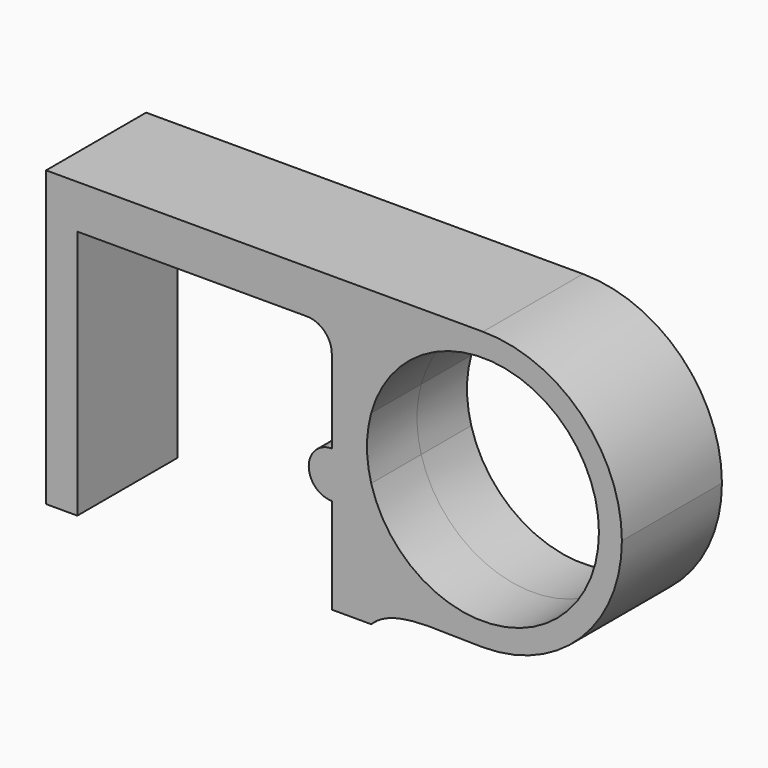
from build123d import *

# Parameters (mm, degrees)
F1_DEPTH = 5


with BuildPart() as f1:
    # F0 (on Front) → F1 (new body, symmetric)
    with BuildSketch(Plane.XZ):
        with BuildLine():
            Line((-24.5694083333, 31.5104130507), (-50.5694083333, 31.5104130507))
            Line((-50.5694083333, 31.5104130507), (-50.5694083333, 8.0104130507))
            Line((-50.5694083333, 8.0104130507), (-48.0694083333, 8.0104130507))
            Line((-48.0694083333, 8.0104130507), (-48.0694083333, 28.0104130507))
            Line((-48.0694083333, 28.0104130507), (-29.7194083333, 28.0104130507))
            ThreePointArc((-29.7194083333, 28.0104130507), (-28.3051947709, 27.424626613), (-27.7194083333, 26.0104130507))
            Line((-27.7194083333, 26.0104130507), (-27.7194083333, 19.3554483443))
            Line((-27.7194083333, 19.3554483443), (-27.7194083333, 15.665377757))
            Line((-27.7194083333, 15.665377757), (-27.7194083333, 8.0104130507))
            Line((-27.7194083333, 8.0104130507), (-24.5694083333, 8.0104130507))
            Line((-24.5694083333, 8.0104130507), (-24.5694083333, 13.8020069146))
            ThreePointArc((-24.5694083333, 13.8020069146), (-26.7411284149, 20.4004295021), (-24.5694083333, 26.9988520897))
            Line((-24.5694083333, 26.9988520897), (-24.5694083333, 31.5104130507))
        make_face()
        with BuildLine():
            ThreePointArc((-15.6311448663, 31.5104130507), (-20.6373094688, 30.3185971969), (-24.5694083333, 26.9988520897))
            Line((-24.5694083333, 26.9988520897), (-24.5694083333, 22.8769333271))
            ThreePointArc((-24.5694083333, 22.8769333271), (-14.3814986476, 29.5908598146), (-6.3561448663, 20.4004295021))
            ThreePointArc((-6.3561448663, 20.4004295021), (-14.3814986476, 11.2099991897), (-24.5694083333, 17.9239256771))
            Line((-24.5694083333, 17.9239256771), (-24.5694083333, 13.8020069146))
            ThreePointArc((-24.5694083333, 13.8020069146), (-20.6371443338, 10.4821784577), (-15.630774911, 9.2904459598))
            ThreePointArc((-15.630774911, 9.2904459598), (-7.7750693624, 12.5446155962), (-4.5211613178, 20.4004295021))
            ThreePointArc((-4.5211613178, 20.4004295021), (-7.7752001603, 28.2563742082), (-15.6311448663, 31.5104130507))
        make_face()
        with BuildLine():
            Line((-24.5694083333, 22.8769333271), (-24.5694083333, 26.9988520897))
            ThreePointArc((-24.5694083333, 26.9988520897), (-26.7411284149, 20.4004295021), (-24.5694083333, 13.8020069146))
            Line((-24.5694083333, 13.8020069146), (-24.5694083333, 17.9239256771))
            ThreePointArc((-24.5694083333, 17.9239256771), (-24.9061448663, 20.4004295021), (-24.5694083333, 22.8769333271))
        make_face()
        with BuildLine():
            ThreePointArc((-15.630774911, 9.2904459598), (-20.6371443338, 10.4821784577), (-24.5694083333, 13.8020069146))
            Line((-24.5694083333, 13.8020069146), (-24.5694083333, 8.0104130507))
            add(Edge.make_bspline(
                [(-24.5694083333, 8.0104130507), (-22.6878308277, 9.9391806871), (-18.7427580517, 9.2241163725), (-15.630774911, 9.2904459598)],
                knots=[0, 0, 0, 0, 9.029820137, 9.029820137, 9.029820137, 9.029820137], degree=3))
        make_face()
        with BuildLine():
            Line((-27.7194083333, 15.665377757), (-27.7194083333, 19.3554483443))
            ThreePointArc((-27.7194083333, 19.3554483443), (-29.564443627, 17.5104130507), (-27.7194083333, 15.665377757))
        make_face()
        with BuildLine():
            Line((-15.6311448663, 31.5104130507), (-24.5694083333, 31.5104130507))
            Line((-24.5694083333, 31.5104130507), (-24.5694083333, 26.9988520897))
            ThreePointArc((-24.5694083333, 26.9988520897), (-20.6373094688, 30.3185971969), (-15.6311448663, 31.5104130507))
        make_face()
    extrude(amount=F1_DEPTH, both=True)


solid = f1.part
